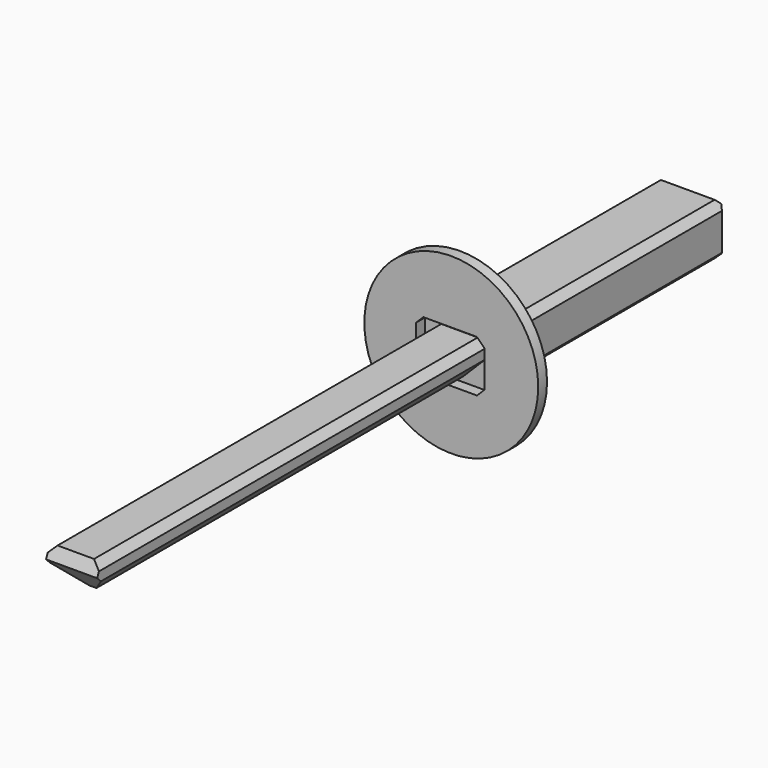
from build123d import *

# Parameters (mm, degrees)
F0_W         = 47.3607815802
F0_H         = 35.7480701059
F1_DEPTH     = 203.2
F2_SIZE      = 5.08
F3_SIZE      = 5.08
F4_R         = 60.2415289401
F5_DEPTH     = 7.62
F6_W         = 35.4304444045
F6_H         = 27.0730024204
F7_DEPTH     = 355.6
F8_SIZE      = 15.24
F9_T1_DEPTH  = 200.9126880875
F10_T1_DEPTH = 357.6371519992
F10_T3_DEPTH = 97.1474137836


# Not quite as in the source:
# - a fillet or chamfer that OpenCascade refuses, or shapes differently, is made with other operations: its cross-section is extruded or revolved along the edge and cut away or added


with BuildPart() as f1:
    # F0 (on Front) → F1 (new body)
    with BuildSketch(Plane.XZ):
        with Locations((-31.144855544, -5.644608289)):
            Rectangle(F0_W, F0_H)
    extrude(amount=-F1_DEPTH)

    # F2
    f2_edges = [f1.edges().sort_by_distance(p)[0] for p in [
        (-7.464465, 101.6, 12.229427),
        (-54.825246, 101.6, 12.229427),
        (-7.464465, 101.6, -23.518643),
    ]]
    chamfer(f2_edges, length=F2_SIZE)

    # F3 (call 1 of 3: OpenCascade refuses the feature's edges together)
    f3_edges = [f1.edges().sort_by_distance(p)[0] for p in [
        (-54.825246, 101.6, -23.518643),
        (-33.684856, 203.2, -23.518643),
        (-54.825246, 203.2, -8.184608),
    ]]
    chamfer(f3_edges, length=F3_SIZE)

    # F3#2 (call 2 of 3)
    f3_2_edges = [f1.edges().sort_by_distance(p)[0] for p in [
        (-31.144856, 203.2, 12.229427),
    ]]
    chamfer(f3_2_edges, length=F3_SIZE)

    # F3#3 (call 3 of 3)
    f3_3_edges = [f1.edges().sort_by_distance(p)[0] for p in [
        (-7.464465, 203.2, -5.644608),
    ]]
    chamfer(f3_3_edges, length=F3_SIZE)

    # F6 (on face) → F7 (join)
    with BuildSketch(Plane.XZ):
        with Locations((-30.7223126292, -6.5321633592)):
            Rectangle(F6_W, F6_H)
    extrude(amount=F7_DEPTH)

    # F8
    f8_edges = [f1.edges().sort_by_distance(p)[0] for p in [
        (-48.437535, -177.8, -20.068665),
        (-13.00709, -177.8, -20.068665),
    ]]
    chamfer(f8_edges, length=F8_SIZE)

    # F9: chamfer of 38.1 on 1 edges, made by hand

    # F9_s2 → F9_t1 (cut)
    with BuildSketch(Plane.YZ.offset(-131.178656673)):
        Polygon((-317.5, -20.0686645694), (-355.6, 18.0313354306), (-355.6, -20.0686645694), align=None)
    extrude(amount=F9_T1_DEPTH, mode=Mode.SUBTRACT)

    # F10: chamfer of 5.08 on 3 edges, made by hand

    # F10_s2 → F10_t1 (cut)
    with BuildSketch(Plane.XZ):
        Polygon((-43.3575348315, 7.004337851), (-48.4375348315, 1.924337851), (-48.4375348315, 7.004337851), align=None)
        Polygon((-13.007090427, 1.924337851), (-18.087090427, 7.004337851), (-13.007090427, 7.004337851), align=None)
    extrude(amount=F10_T1_DEPTH, mode=Mode.SUBTRACT)

    # F10_s4 → F10_t3 (cut)
    with BuildSketch(Plane.YZ.offset(-79.296019521)):
        Polygon((-332.3087975235, 7.004337851), (-335.9008999719, -1.6677645975), (-344.5730024204, 7.004337851), align=None)
    extrude(amount=F10_T3_DEPTH, mode=Mode.SUBTRACT)


with BuildPart() as f5:
    # F4 (on face) → F5 (new body)
    with BuildSketch(Plane.XZ):
        with Locations((-30.3635057062, -4.4609890319)):
            Circle(F4_R)
        Polygon((-54.8252463341, -18.438643342), (-54.8252463341, 7.149426764), (-49.7452463341, 12.229426764), (-12.5444647539, 12.229426764), (-7.4644647539, 7.149426764), (-7.4644647539, -18.438643342), (-12.5444647539, -23.518643342), (-49.7452463341, -23.518643342), align=None, mode=Mode.SUBTRACT)
    extrude(amount=F5_DEPTH)


solid = Compound([f1.part, f5.part])
